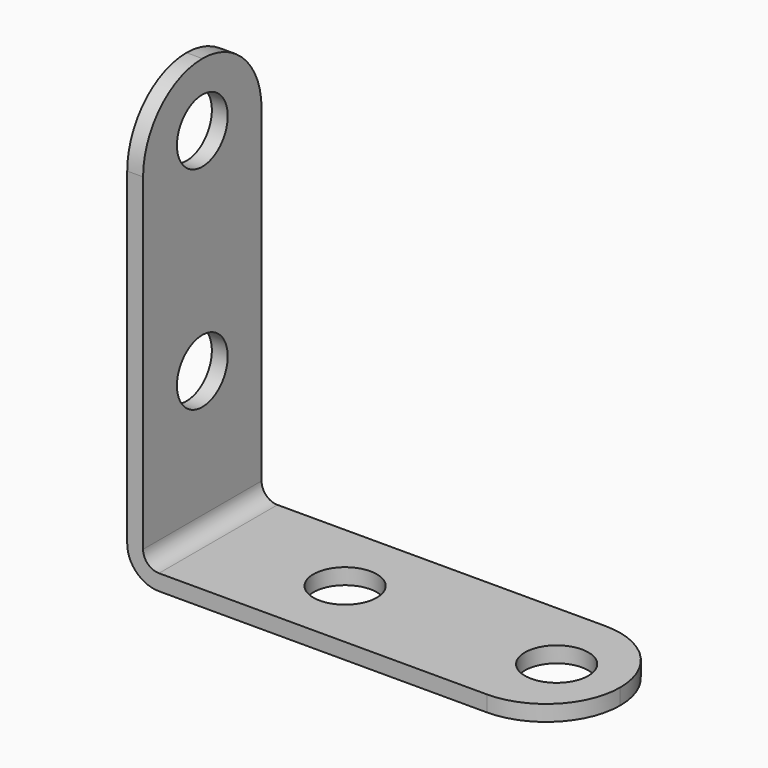
from build123d import *

# Parameters (mm, degrees)
F1_DEPTH = 14
F2_R     = 6.99999
F3_R     = 3
F4_DEPTH = 25
F5_R     = 3
F6_DEPTH = 25


# Not quite as in the source:
# - a fillet or chamfer is up to 0.001 mm smaller than in the source, because OpenCascade refuses the exact size


with BuildPart() as f1:
    # F0 (on Front) → F1 (new body)
    with BuildSketch(Plane.XZ):
        with BuildLine():
            Line((3, 0), (41, 0))
            Line((41, 0), (41, 1.5))
            Line((41, 1.5), (3, 1.5))
            ThreePointArc((3, 1.5), (1.9393398282, 1.9393398282), (1.5, 3))
            Line((1.5, 3), (1.5, 41))
            Line((1.5, 41), (0, 41))
            Line((0, 41), (0, 3))
            ThreePointArc((0, 3), (0.8786796564, 0.8786796564), (3, 0))
        make_face()
    extrude(amount=F1_DEPTH)

    # F2 (radius 7 in the source; OpenCascade refuses exactly that, so slightly less here)
    f2_edges = [f1.edges().sort_by_distance(p)[0] for p in [
        (41, 0, 0.75),
        (41, -14, 0.75),
        (0.75, 0, 41),
        (0.75, -14, 41),
    ]]
    fillet(f2_edges, radius=F2_R)

    # F3 (on face) → F4 (cut)
    with BuildSketch(Plane(origin=(0, 0, 0), x_dir=(0, -1, 0), z_dir=(-1, 0, 0))):
        with Locations((7, 15)):
            Circle(F3_R)
        with Locations((7, 35)):
            Circle(F3_R)
    extrude(amount=-F4_DEPTH, mode=Mode.SUBTRACT)

    # F5 (on face) → F6 (cut)
    with BuildSketch(Plane(origin=(0, 0, 0), x_dir=(1, 0, 0), z_dir=(0, 0, -1))):
        with Locations((35, 7)):
            Circle(F5_R)
        with Locations((15, 7)):
            Circle(F5_R)
    extrude(amount=-F6_DEPTH, mode=Mode.SUBTRACT)


solid = f1.part
